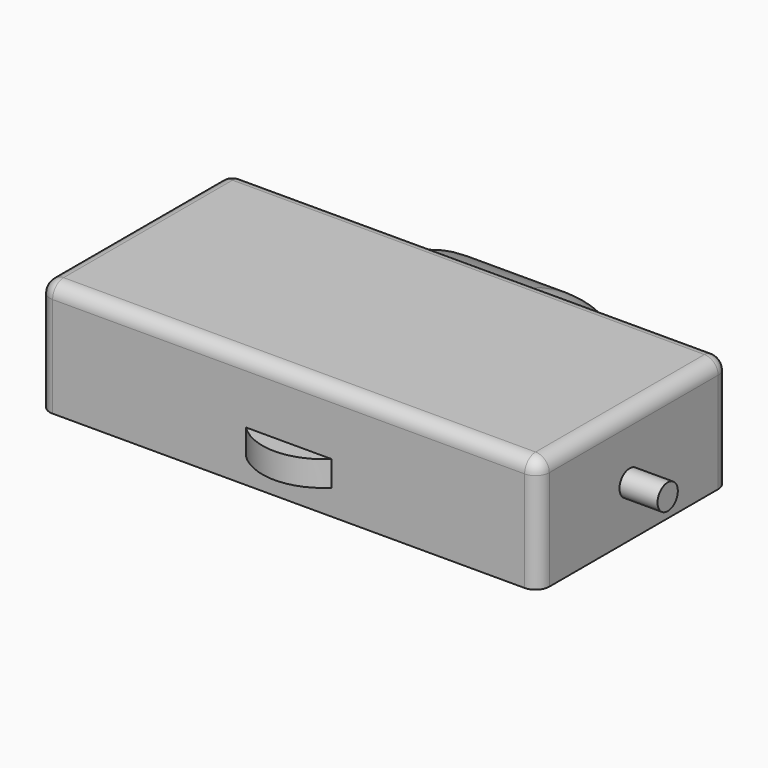
from build123d import *

# Parameters (mm, degrees)
F0_W      = 62.5094
F0_H      = 29.845
F1_DEPTH  = 14.2875
F4_DEPTH  = 3.175
F5_R      = 0.3175
F6_R      = 1.7145
F7_W      = 56.1594
F7_H      = 23.495
F8_DEPTH  = 10.1
F9_R      = 1.7145
F10_R     = 1.5875
F11_DEPTH = 4.7625
F12_R     = 1.5875
F13_DEPTH = 4.7625
F15_DEPTH = 8
F16_R     = 1.7145
F17_R     = 1.5875
F18_DEPTH = 1.7145
F19_R     = 1.5875
F20_DEPTH = 1.7145


with BuildPart() as f1:
    # F0 (on Top) → F1 (new body)
    with BuildSketch(Plane.XY):
        Rectangle(F0_W, F0_H)
    extrude(amount=F1_DEPTH)

    # F6
    f6_edges = [f1.edges().sort_by_distance(p)[0] for p in [
        (-31.2547, -14.9225, 7.14375),
        (31.2547, -14.9225, 7.14375),
        (31.2547, 14.9225, 7.14375),
        (-31.2547, 14.9225, 7.14375),
        (0, 14.9225, 14.2875),
        (-31.2547, 0, 14.2875),
        (0, -14.9225, 14.2875),
        (31.2547, 0, 14.2875),
    ]]
    fillet(f6_edges, radius=F6_R)

    # F7 (on face) → F8 (cut)
    with BuildSketch(Plane(origin=(0, 0, 0), x_dir=(1, 0, 0), z_dir=(0, 0, -1))):
        Rectangle(F7_W, F7_H)
    extrude(amount=-F8_DEPTH, mode=Mode.SUBTRACT)

    # F9
    f9_edges = [f1.edges().sort_by_distance(p)[0] for p in [
        (-28.0797, 11.7475, 5.05),
        (-28.0797, -11.7475, 5.05),
        (28.0797, -11.7475, 5.05),
        (28.0797, 11.7475, 5.05),
    ]]
    fillet(f9_edges, radius=F9_R)

    # F10 (on face) → F11 (join)
    with BuildSketch(Plane.YZ.offset(31.2547)):
        with Locations((-0.635, 6.35)):
            Circle(F10_R)
    extrude(amount=F11_DEPTH)

    # F12 (on face) → F13 (join)
    with BuildSketch(Plane(origin=(-31.2547, 0, 0), x_dir=(0, -1, 0), z_dir=(-1, 0, 0))):
        with Locations((-0.635, 6.35)):
            Circle(F12_R)
    extrude(amount=F13_DEPTH)

    # F14 (on Right) → F15 (join, symmetric)
    with BuildSketch(Plane.YZ):
        with BuildLine():
            Line((11.938, 14.2875), (11.938, 0))
            Line((11.938, 0), (19.938, 0))
            Line((19.938, 0), (19.938, -5))
            Line((19.938, -5), (29.938, -5))
            Line((29.938, -5), (29.938, 0))
            ThreePointArc((29.938, 0), (22.5268828144, 9.1454921283), (11.938, 14.2875))
        make_face()
    extrude(amount=F15_DEPTH, both=True)

    # F16
    f16_edges = [f1.edges().sort_by_distance(p)[0] for p in [
        (8, 23.613613, 8.235594),
        (-8, 23.613613, 8.235594),
    ]]
    fillet(f16_edges, radius=F16_R)

    # F17 (on face) → F18 (join)
    with BuildSketch(Plane.YZ.offset(8)):
        with Locations((24.938, -1.825)):
            Circle(F17_R)
    extrude(amount=F18_DEPTH)

    # F19 (on face) → F20 (join)
    with BuildSketch(Plane(origin=(-8, 0, 0), x_dir=(0, -1, 0), z_dir=(-1, 0, 0))):
        with Locations((-24.9487477744, -1.825)):
            Circle(F19_R)
    extrude(amount=F20_DEPTH)


with BuildPart() as f4:
    # F3 (on offset) → F4 (new body)
    with BuildSketch(Plane.XY.offset(3.175)):
        with BuildLine():
            Line((5.8547, -14.3758933991), (-5.8547, -14.3758933991))
            ThreePointArc((-5.8547, -14.3758933991), (0, -17.1187130754), (5.8547, -14.3758933991))
        make_face()
    extrude(amount=F4_DEPTH)

    # F5
    f5_edges = [f4.edges().sort_by_distance(p)[0] for p in [
        (-5.8547, -14.375893, 4.7625),
        (0, -14.375893, 6.35),
        (0, -14.375893, 3.175),
        (5.8547, -14.375893, 4.7625),
    ]]
    fillet(f5_edges, radius=F5_R)


solid = Compound([f1.part, f4.part])
